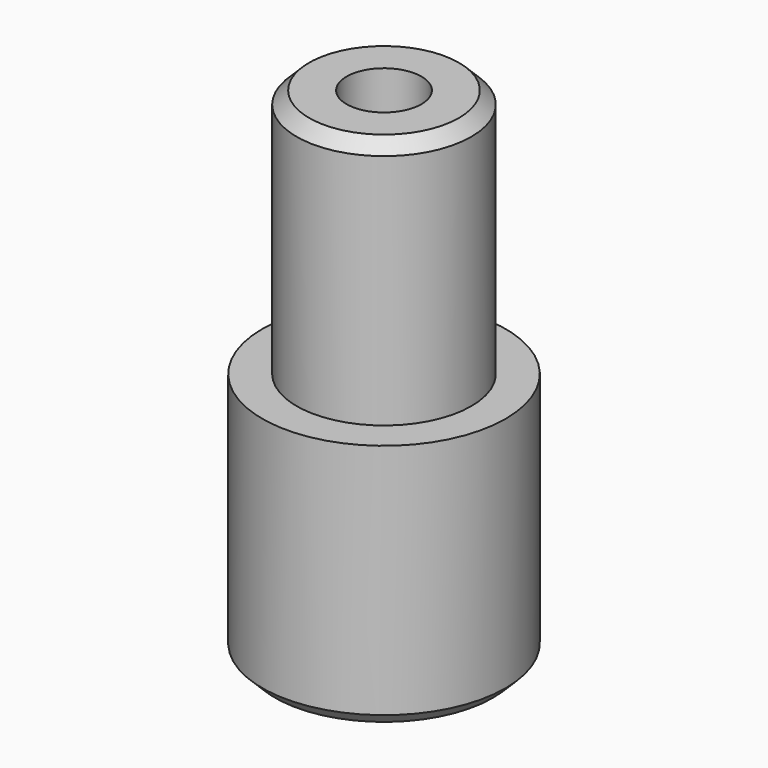
from build123d import *

# Parameters (mm, degrees)
F0_R     = 7
F0_R_2   = 3
F1_DEPTH = 20
F0_R_3   = 9.75
F2_DEPTH = 20
F3_R     = 4
F3_R_2   = 3
F4_DEPTH = 10
F5_SIZE  = 0.99999


# Not quite as in the source:
# - a fillet or chamfer is up to 0.001 mm smaller than in the source, because OpenCascade refuses the exact size


with BuildPart() as f1:
    # F0 (on Top) → F1 (new body)
    with BuildSketch(Plane.XY):
        Circle(F0_R)
        Circle(F0_R_2, mode=Mode.SUBTRACT)
    extrude(amount=F1_DEPTH)

    # F0 (on Top) → F2 (join)
    with BuildSketch(Plane.XY):
        Circle(F0_R_3)
        Circle(F0_R, mode=Mode.SUBTRACT)
        Circle(F0_R)
        Circle(F0_R_2, mode=Mode.SUBTRACT)
    extrude(amount=-F2_DEPTH)

    # F3 (on face) → F4 (cut)
    with BuildSketch(Plane(origin=(0, 0, -20), x_dir=(1, 0, 0), z_dir=(0, 0, -1))):
        Circle(F3_R)
        Circle(F3_R_2, mode=Mode.SUBTRACT)
    extrude(amount=-F4_DEPTH, mode=Mode.SUBTRACT)

    # F5 (size 1 in the source; OpenCascade refuses exactly that, so slightly less here)
    f5_edges = [f1.edges().sort_by_distance(p)[0] for p in [
        (-9.75, 0, -20),
        (-7, 0, 20),
        (-3, 0, -10),
    ]]
    chamfer(f5_edges, length=F5_SIZE)


solid = f1.part
